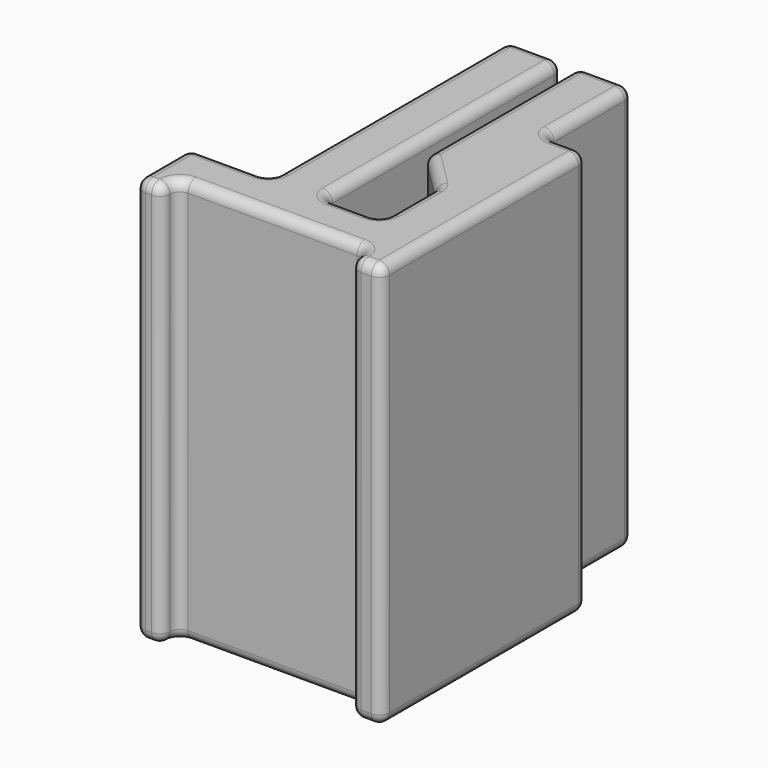
from build123d import *

# Parameters (mm, degrees)
F1_DEPTH = 30
F2_W     = 14
F2_H     = 30
F3_DEPTH = 1.5
F4_F1_R  = 0.75
F4_F2_R  = 0.7499


# Not quite as in the source:
# - a fillet or chamfer is up to 0.001 mm smaller than in the source, because OpenCascade refuses the exact size


with BuildPart() as f1:
    # F0 (on Top) → F1 (new body)
    with BuildSketch(Plane.XY):
        Polygon((16, 14), (16, -8), (10, -8), (10, -13), (28.2, -13), (28.2, 6), (25.2, 6), (25.2, 14), (21.2, 14), (21.2, 0), (24.2, -3), (24.2, -8), (20, -8), (20, 14), align=None)
    extrude(amount=F1_DEPTH)

    # F2 (on face) → F3 (cut)
    with BuildSketch(Plane.XZ.offset(13)):
        with Locations((18.95, 15)):
            Rectangle(F2_W, F2_H)
    extrude(amount=-F3_DEPTH, mode=Mode.SUBTRACT)

    # F4: fillet of radius 0.75 on 50 edges, made by hand

    # F4_f1
    f4_f1_edges = [f1.edges().sort_by_distance(p)[0] for p in [
        (16, -8, 15),
        (24.2, -8, 15),
        (20, -8, 15),
        (25.95, -11.5, 15),
        (11.95, -11.5, 15),
        (25.2, 6, 15),
        (24.2, -3, 15),
    ]]
    fillet(f4_f1_edges, radius=F4_F1_R)

    # F4_f2 (radius 0.75 in the source; OpenCascade refuses exactly that, so slightly less here)
    f4_f2_edges = [f1.edges().sort_by_distance(p)[0] for p in [
        (21.2, 14, 15),
        (10, -8, 15),
        (10, -10.5, 30),
        (10, -10.5, 0),
        (12.625, -8, 30),
        (16, 3.375, 30),
        (16, 14, 15),
        (16, 3.375, 0),
        (23.2, 14, 0),
        (20, 14, 15),
        (20, 3.375, 30),
        (21.2, 7, 30),
        (22.1, -8, 30),
        (21.2, 7, 0),
        (20, 3.375, 0),
        (23.2, 14, 30),
        (18, 14, 30),
        (18, 14, 0),
        (10, -13, 15),
        (11.95, -13, 15),
        (18.95, -11.5, 30),
        (28.2, -13, 15),
        (28.2, -3.5, 30),
        (25.95, -13, 15),
        (18.95, -11.5, 0),
        (28.2, -3.5, 0),
        (25.95, -12.625, 0),
        (25.95, -12.625, 30),
        (11.95, -12.625, 30),
        (11.95, -12.625, 0),
        (10.975, -13, 0),
        (10.975, -13, 30),
        (27.075, -13, 30),
        (27.075, -13, 0),
        (28.2, 6, 15),
        (25.2, 14, 15),
        (25.2, 10.375, 30),
        (27.075, 6, 30),
        (27.075, 6, 0),
        (25.2, 10.375, 0),
        (21.2, 0, 15),
        (22.5901650429, -1.3901650429, 0),
        (22.5901650429, -1.3901650429, 30),
        (24.1429096494, -3.0236475975, 30),
        (24.1429096494, -3.0236475975, 0),
        (25.4196699141, 6.2196699141, 0),
        (25.4196699141, 6.2196699141, 30),
        (12.1696699141, -11.7196699141, 0),
        (12.1696699141, -11.7196699141, 30),
        (25.7303300859, -11.7196699141, 30),
        (25.7303300859, -11.7196699141, 0),
        (20.2196699141, -7.7803300859, 0),
        (23.9803300859, -7.7803300859, 30),
        (20.2196699141, -7.7803300859, 30),
        (15.7803300859, -7.7803300859, 0),
        (15.7803300859, -7.7803300859, 30),
    ]]
    fillet(f4_f2_edges, radius=F4_F2_R)


solid = f1.part
